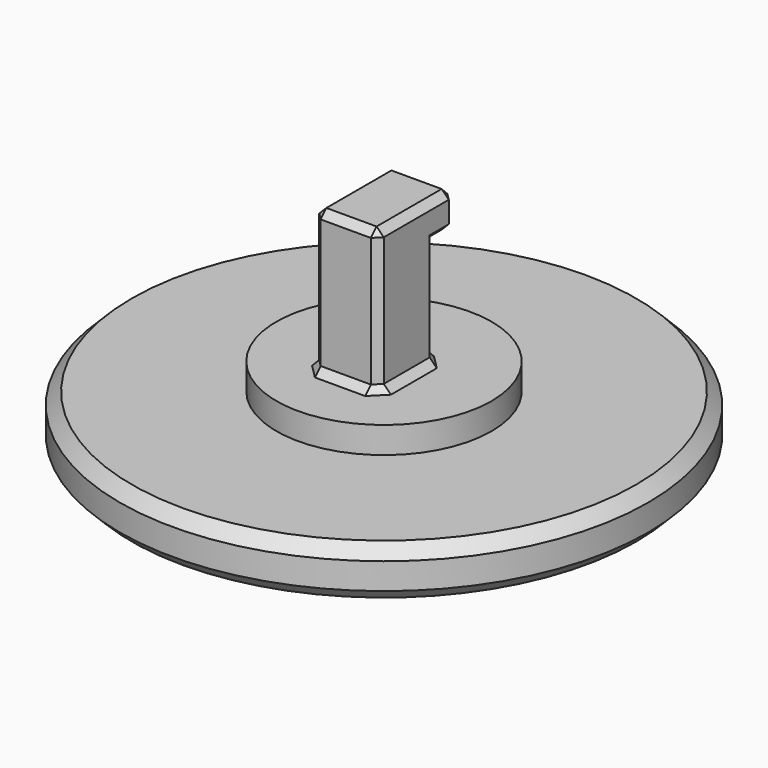
from build123d import *

# Parameters (mm, degrees)
F0_R     = 11.05
F1_DEPTH = 2.1
F2_R     = 4.5
F3_DEPTH = 1.11
F6_DEPTH = 6
F7_W     = 2.7
F7_H     = 1.5
F8_DEPTH = 1
F9_SIZE  = 0.3
F10_SIZE = 0.5


# Not quite as in the source:
# - two fillets or chamfers of one size are made in one step


with BuildPart() as f1:
    # F0 (on Top) → F1 (new body)
    with BuildSketch(Plane.XY):
        Circle(F0_R)
    extrude(amount=F1_DEPTH)

    # F2 (on face) → F3 (join)
    with BuildSketch(Plane.XY.offset(2.1)):
        Circle(F2_R)
    extrude(amount=F3_DEPTH)

    # F5 (on face) → F6 (join)
    with BuildSketch(Plane.XY.offset(3.21)):
        Polygon((-1.35, -2), (1.35, -2), (1.35, 0), (1.35, 1), (-1.35, 1), (-1.35, 0), align=None)
    extrude(amount=F6_DEPTH)

    # F7 (on face) → F8 (join)
    with BuildSketch(Plane(origin=(0, 1, 0), x_dir=(-1, 0, 0), z_dir=(0, 1, 0))):
        with Locations((0, 8.46)):
            Rectangle(F7_W, F7_H)
    extrude(amount=F8_DEPTH)

    # F9
    f9_edges = [f1.edges().sort_by_distance(p)[0] for p in [
        (-1.35, -2, 6.21),
        (1.35, -2, 6.21),
        (1.35, 1, 5.46),
        (-1.35, 1, 5.46),
        (1.35, 1.5, 7.71),
        (-1.35, 1.5, 7.71),
        (0, 2, 7.71),
        (1.35, 2, 8.46),
        (-1.35, 2, 8.46),
        (0, 2, 9.21),
        (1.35, 0, 9.21),
        (-1.35, 0, 9.21),
        (0, -2, 9.21),
        (-1.35, -0.5, 3.21),
        (0, -2, 3.21),
        (1.35, -0.5, 3.21),
        (0, 1, 3.21),
    ]]
    chamfer(f9_edges, length=F9_SIZE)

    # F10
    f10_edges = [f1.edges().sort_by_distance(p)[0] for p in [
        (-11.05, 0, 0),
        (-11.05, 0, 2.1),
    ]]
    chamfer(f10_edges, length=F10_SIZE)


solid = f1.part
